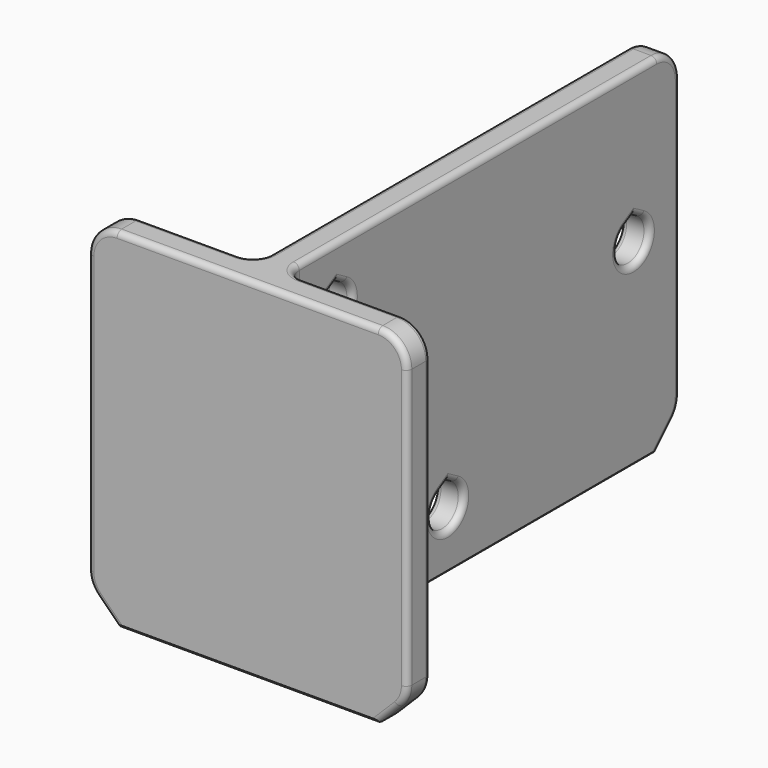
from build123d import *

# Parameters (mm, degrees)
F0_W          = 85
F0_H          = 60
F1_DEPTH      = 5
F2_W          = 55
F2_H          = 60
F3_DEPTH      = 5
F5_DEPTH      = 5
F6_R          = 3
F7_SIZE       = 5
F8_R          = 5
F9_R          = 1
F10_T1_DEPTH  = 16.8716279316
F10_T3_DEPTH  = 76.8716279316
F10_T5_DEPTH  = 16.8716279316
F10_T7_DEPTH  = 44.7432558632
F10_T10_ANGLE = 90
F10_T12_ANGLE = 90


# Not quite as in the source:
# - a fillet or chamfer that OpenCascade refuses, or shapes differently, is made with other operations: its cross-section is extruded or revolved along the edge and cut away or added


with BuildPart() as f1:
    # F0 (on Right) → F1 (new body)
    with BuildSketch(Plane.YZ):
        with Locations((7.5, 30)):
            Rectangle(F0_W, F0_H)
    extrude(amount=F1_DEPTH)

    # F2 (on face) → F3 (join)
    with BuildSketch(Plane.XZ.offset(35)):
        with Locations((2.5, 30)):
            Rectangle(F2_W, F2_H)
    extrude(amount=F3_DEPTH)

    # F4 (on face) → F5 (cut, through all)
    with BuildSketch(Plane.YZ.offset(5)):
        with BuildLine():
            Line((-24, 54.0414518843), (-25.75, 53.0310889132))
            ThreePointArc((-25.75, 53.0310889132), (-24, 46.5), (-22.25, 53.0310889132))
            Line((-22.25, 53.0310889132), (-24, 54.0414518843))
        make_face()
        with BuildLine():
            Line((0, 14.0414518843), (-1.75, 13.0310889132))
            ThreePointArc((-1.75, 13.0310889132), (0, 6.5), (1.75, 13.0310889132))
            Line((1.75, 13.0310889132), (0, 14.0414518843))
        make_face()
        with BuildLine():
            Line((40, 38.0414518843), (38.25, 37.0310889132))
            ThreePointArc((38.25, 37.0310889132), (40, 30.5), (41.75, 37.0310889132))
            Line((41.75, 37.0310889132), (40, 38.0414518843))
        make_face()
    extrude(amount=-F5_DEPTH, mode=Mode.SUBTRACT)

    # F6
    f6_edges = [f1.edges().sort_by_distance(p)[0] for p in [
        (5, -35, 30),
        (0, -35, 30),
    ]]
    fillet(f6_edges, radius=F6_R)

    # F7
    f7_edges = [f1.edges().sort_by_distance(p)[0] for p in [
        (30, -37.5, 0),
        (2.5, 50, 0),
        (-25, -37.5, 0),
    ]]
    chamfer(f7_edges, length=F7_SIZE)

    # F8
    f8_edges = [f1.edges().sort_by_distance(p)[0] for p in [
        (30, -37.5, 60),
        (-25, -37.5, 60),
        (2.5, 50, 60),
        (30, -37.5, 5),
        (2.5, 50, 5),
        (-25, -37.5, 5),
    ]]
    fillet(f8_edges, radius=F8_R)

    # F9
    f9_edges = [f1.edges().sort_by_distance(p)[0] for p in [
        (30, -35, 31.035534),
        (-25, -35, 31.035534),
        (30, -40, 31.035534),
        (2.5, -25.75, 53.031089),
        (2.5, -22.25, 53.031089),
        (5, -24, 46.5),
        (0, -24, 46.5),
        (2.5, -1.75, 13.031089),
        (2.5, 1.75, 13.031089),
        (5, 0, 6.5),
        (0, 0, 6.5),
        (2.5, 38.25, 37.031089),
        (2.5, 41.75, 37.031089),
        (5, 40, 30.5),
        (0, 40, 30.5),
        (-23.535534, -35, 58.535534),
        (-24.619398, -35, 5.157651),
        (-11.5, -35, 60),
        (-21.767767, -35, 1.767767),
        (-25, -40, 31.035534),
        (-23.535534, -40, 58.535534),
        (-24.619398, -40, 5.157651),
        (-0.87868, -34.12132, 60),
        (2.5, -40, 60),
        (0, 6.5, 60),
        (16.5, -35, 60),
        (5, 6.5, 60),
        (5.87868, -34.12132, 60),
        (-21.767767, -40, 1.767767),
        (28.535534, -40, 58.535534),
        (26.767767, -40, 1.767767),
        (29.619398, -40, 5.157651),
        (0, 50, 31.035534),
        (0, 49.619398, 5.157651),
        (0, 48.535534, 58.535534),
        (0, 46.767767, 1.767767),
        (0, 0.875, 13.53627),
        (0, -0.875, 13.53627),
        (0, -23.125, 53.53627),
        (0, -24.875, 53.53627),
        (0, 39.125, 37.53627),
        (0, 40.875, 37.53627),
        (28.535534, -35, 58.535534),
        (5, 48.535534, 58.535534),
        (29.619398, -35, 5.157651),
        (26.767767, -35, 1.767767),
        (5, 50, 31.035534),
        (5, 49.619398, 5.157651),
        (5, 46.767767, 1.767767),
        (5, 0.875, 13.53627),
        (5, -0.875, 13.53627),
        (5, -23.125, 53.53627),
        (5, -24.875, 53.53627),
        (5, 39.125, 37.53627),
        (5, 40.875, 37.53627),
    ]]
    fillet(f9_edges, radius=F9_R)

    # F10: chamfer of 0.5 on 7 edges, made by hand

    # F10_s2 → F10_t1 (cut)
    with BuildSketch(Plane.YZ.offset(-19.8716279316)):
        Polygon((-35, 0.5), (-35.5, 0), (-35, 0), align=None)
    extrude(amount=F10_T1_DEPTH, mode=Mode.SUBTRACT)

    # F10_s4 → F10_t3 (cut)
    with BuildSketch(Plane.XZ.offset(-44.8716279316)):
        Polygon((0.5, 0), (0, 0.5), (0, 0), align=None)
        Polygon((4.5, 0), (5, 0.5), (5, 0), align=None)
    extrude(amount=F10_T3_DEPTH, mode=Mode.SUBTRACT)

    # F10_s6 → F10_t5 (cut)
    with BuildSketch(Plane.YZ.offset(8)):
        Polygon((-35.5, 0), (-35, 0.5), (-35, 0), align=None)
    extrude(amount=F10_T5_DEPTH, mode=Mode.SUBTRACT)

    # F10_s8 → F10_t7 (cut)
    with BuildSketch(Plane.YZ.offset(-19.8716279316)):
        Polygon((-39.5, 0), (-40, 0.5), (-40, 0), align=None)
    extrude(amount=F10_T7_DEPTH, mode=Mode.SUBTRACT)

    # F10_s9 → F10_t10 (revolve, cut)
    with BuildSketch(Plane.YZ.offset(-3)):
        Polygon((-35, 0.5), (-35.5, 0), (-35, 0), align=None)
    revolve(axis=Axis((-3, -32, 0), (0, 0, 1)), revolution_arc=F10_T10_ANGLE, mode=Mode.SUBTRACT)

    # F10_s11 → F10_t12 (revolve, cut)
    with BuildSketch(Plane.XZ.offset(32)):
        Polygon((4.5, 0), (5, 0.5), (5, 0), align=None)
    revolve(axis=Axis((8, -32, 0), (0, 0, 1)), revolution_arc=F10_T12_ANGLE, mode=Mode.SUBTRACT)


solid = f1.part
